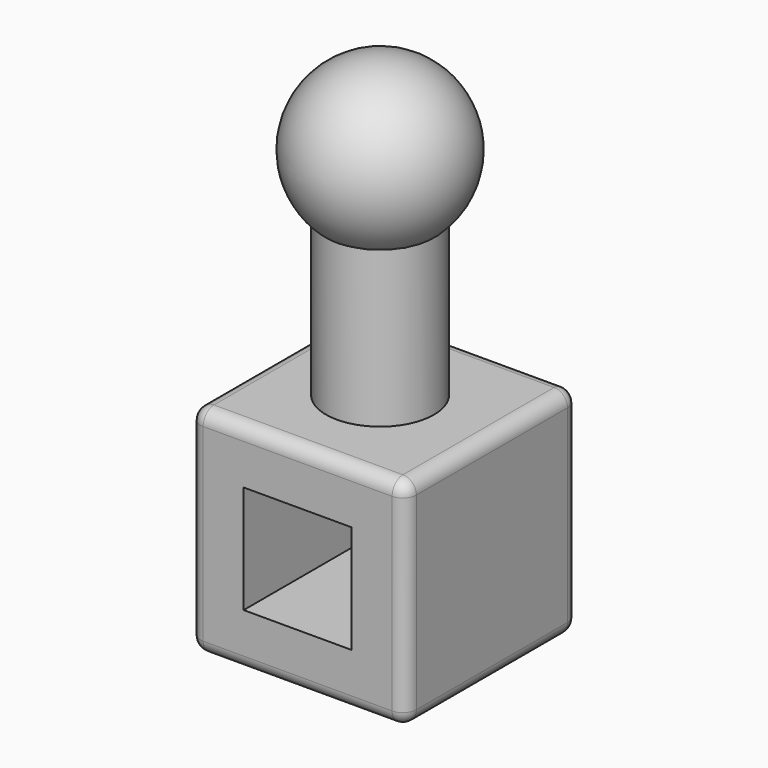
from build123d import *

# Parameters (mm, degrees)
F0_W     = 101.6
F0_H     = 101.6
F1_DEPTH = 101.6
F2_R     = 25.4
F3_DEPTH = 101.6
F6_W     = 50.8
F6_H     = 50.8
F7_DEPTH = 101.6
F8_R     = 6.35


# Not quite as in the source:
# - a feature names something its author has since deleted; it is built from what else it names


with BuildPart() as f1:
    # F0 (on Front) → F1 (new body)
    with BuildSketch(Plane.XZ):
        with Locations((1.857098192, 6.5613021186)):
            Rectangle(F0_W, F0_H)
    extrude(amount=F1_DEPTH)

    # F2 (on face) → F3 (join)
    with BuildSketch(Plane.XY.offset(57.3613021186)):
        with Locations((0, -50.8)):
            Circle(F2_R)
    extrude(amount=F3_DEPTH)

    # F6 (on face) → F7 (cut)
    with BuildSketch(Plane.XZ.offset(101.6)):
        with Locations((1.857098192, 6.5613021186)):
            Rectangle(F6_W, F6_H)
    extrude(amount=-F7_DEPTH, mode=Mode.SUBTRACT)

    # F8
    f8_edges = [f1.edges().sort_by_distance(p)[0] for p in [
        (1.857098, -101.6, 57.361302),
        (52.657098, -101.6, 6.561302),
        (1.857098, -101.6, -44.238698),
        (-48.942902, -101.6, 6.561302),
        (-48.942902, -50.8, 57.361302),
        (1.857098, 0, 57.361302),
        (52.657098, -50.8, 57.361302),
        (52.657098, -50.8, -44.238698),
        (52.657098, 0, 6.561302),
        (1.857098, 0, -44.238698),
        (-48.942902, -50.8, -44.238698),
        (-48.942902, 0, 6.561302),
    ]]
    fillet(f8_edges, radius=F8_R)


with BuildPart() as f5:
    # F4 (on face) → F5 (revolve)
    with BuildSketch(Plane.XY.offset(158.9613021186)):
        with BuildLine():
            Line((0, -25.4), (0, -12.7))
            ThreePointArc((0, -12.7), (-38.1, -50.8), (0, -88.9))
            Line((0, -88.9), (0, -76.2))
            ThreePointArc((0, -76.2), (-25.4, -50.8), (0, -25.4))
        make_face()
        with BuildLine():
            Line((0, -76.2), (0, -25.4))
            ThreePointArc((0, -25.4), (-25.4, -50.8), (0, -76.2))
        make_face()
    revolve(axis=Axis((0, -50.8, 158.9613021186), (0, -1, 0)))


solid = Compound([f1.part, f5.part])
